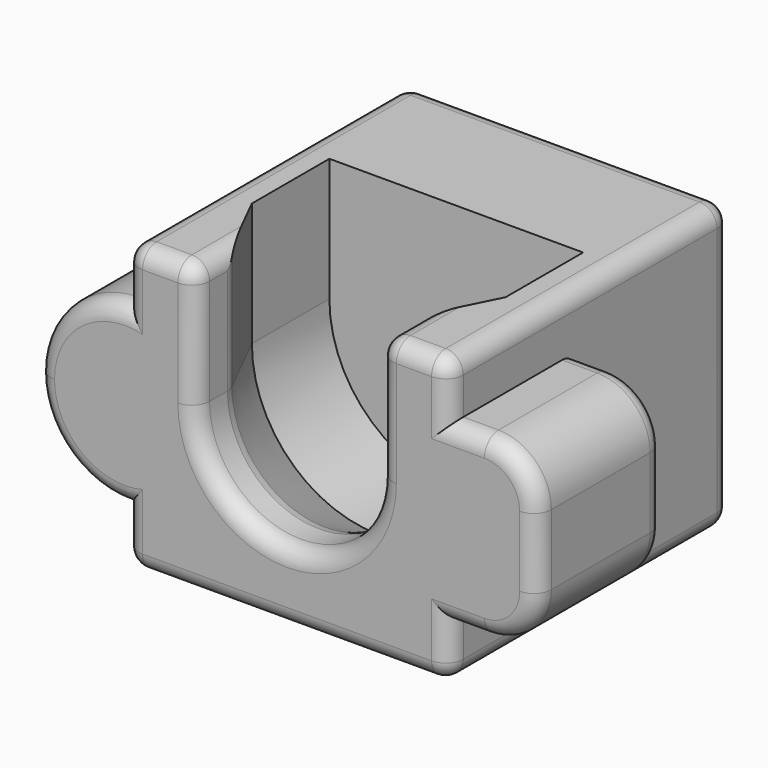
from build123d import *

# Parameters (mm, degrees)
F1_ANGLE = 180
F3_DEPTH = 14
F4_DEPTH = 7
F6_DEPTH = 14
F7_DEPTH = 5
F5_W     = 5
F5_H     = 10
F8_DEPTH = 6
F9_R     = 1


with BuildPart() as f1:
    # F0 (on Top) → F1 (revolve)
    with BuildSketch(Plane.XY):
        Polygon((-9.2, 14), (-9.2, 0), (-5.2, 0), (-5.2, 2.5), (-7.2, 6.5), (-7.2, 12), (0, 12), (0, 14), align=None)
    revolve(axis=Axis((0, -5.2679181099, 0), (0, -1, 0)), revolution_arc=F1_ANGLE)

    # F2 (on face) → F3 (join, through all)
    with BuildSketch(Plane(origin=(0, 14, 0), x_dir=(-1, 0, 0), z_dir=(0, 1, 0))):
        with BuildLine():
            ThreePointArc((-7.9e-09, -9.2), (-6.5053823897, -6.5053823841), (-9.2, 0))
            Line((-9.2, 0), (-9.2, -9.2))
            Line((-9.2, -9.2), (-7.9e-09, -9.2))
        make_face()
        with BuildLine():
            ThreePointArc((9.2, 0), (6.5053823841, -6.5053823897), (-7.9e-09, -9.2))
            Line((-7.9e-09, -9.2), (9.2, -9.2))
            Line((9.2, -9.2), (9.2, 0))
        make_face()
    extrude(amount=-F3_DEPTH)

    # F4 (add): a face of the model
    f4_faces = [f1.faces().sort_by_distance(p)[0] for p in [
        (-8.9687944637, 7, 0),
    ]]
    extrude(f4_faces, amount=F4_DEPTH)

    # F5 (on face) → F6 (join, through all)
    with BuildSketch(Plane(origin=(0, 14, 0), x_dir=(-1, 0, 0), z_dir=(0, 1, 0))):
        with BuildLine():
            ThreePointArc((9.2, -6.1), (12.7355339059, -4.6355339059), (14.2, -1.1))
            ThreePointArc((14.2, -1.1), (12.7355339059, 2.4355339059), (9.2, 3.9))
            Line((9.2, 3.9), (9.2, -6.1))
        make_face()
        with BuildLine():
            Line((-9.2, -6.1), (-9.2, 3.9))
            Line((-9.2, 3.9), (-11.2, 3.9))
            ThreePointArc((-11.2, 3.9), (-13.3213203436, 3.0213203436), (-14.2, 0.9))
            Line((-14.2, 0.9), (-14.2, -3.1))
            ThreePointArc((-14.2, -3.1), (-13.3213203436, -5.2213203436), (-11.2, -6.1))
            Line((-11.2, -6.1), (-9.2, -6.1))
        make_face()
    extrude(amount=-F6_DEPTH)

    # F5 (on face) → F7 (cut)
    with BuildSketch(Plane(origin=(0, 14, 0), x_dir=(-1, 0, 0), z_dir=(0, 1, 0))):
        with BuildLine():
            ThreePointArc((9.2, -6.1), (12.7355339059, -4.6355339059), (14.2, -1.1))
            ThreePointArc((14.2, -1.1), (12.7355339059, 2.4355339059), (9.2, 3.9))
            Line((9.2, 3.9), (9.2, -6.1))
        make_face()
        with BuildLine():
            Line((-9.2, -6.1), (-9.2, 3.9))
            Line((-9.2, 3.9), (-11.2, 3.9))
            ThreePointArc((-11.2, 3.9), (-13.3213203436, 3.0213203436), (-14.2, 0.9))
            Line((-14.2, 0.9), (-14.2, -3.1))
            ThreePointArc((-14.2, -3.1), (-13.3213203436, -5.2213203436), (-11.2, -6.1))
            Line((-11.2, -6.1), (-9.2, -6.1))
        make_face()
    extrude(amount=-F7_DEPTH, mode=Mode.SUBTRACT)

    # F5 (on face) → F8 (join)
    with BuildSketch(Plane(origin=(0, 14, 0), x_dir=(-1, 0, 0), z_dir=(0, 1, 0))):
        with BuildLine():
            Line((9.2, -6.1), (9.2, 3.9))
            ThreePointArc((9.2, 3.9), (4.2, -1.1), (9.2, -6.1))
        make_face()
        with BuildLine():
            ThreePointArc((9.2, -6.1), (4.2, -1.1), (9.2, 3.9))
            Line((9.2, 3.9), (9.2, 7))
            Line((9.2, 7), (-9.2, 7))
            Line((-9.2, 7), (-9.2, 3.9))
            Line((-9.2, 3.9), (-4.2, 3.9))
            Line((-4.2, 3.9), (-4.2, -6.1))
            Line((-4.2, -6.1), (-9.2, -6.1))
            Line((-9.2, -6.1), (-9.2, -9.2))
            Line((-9.2, -9.2), (9.2, -9.2))
            Line((9.2, -9.2), (9.2, -6.1))
        make_face()
        with Locations((-6.7, -1.1)):
            Rectangle(F5_W, F5_H)
    extrude(amount=F8_DEPTH)

    # F9
    f9_edges = [f1.edges().sort_by_distance(p)[0] for p in [
        (9.2, 10, 7),
        (-9.2, 10, 7),
        (9.2, 10, -9.2),
        (-9.2, 10, -9.2),
        (-7.2, 0, 7),
        (9.2, 0, 5.45),
        (9.2, 0, -7.65),
        (-9.2, 0, -7.65),
        (-9.2, 0, 5.45),
        (0, 0, -9.2),
        (0, 0, -5.2),
        (-5.2, 0, 3.5),
        (-14.2, 0, -1.1),
        (10.2, 0, -6.1),
        (13.32132, 0, -5.22132),
        (14.2, 0, -1.1),
        (13.32132, 0, 3.02132),
        (10.2, 0, 3.9),
        (7.2, 0, 7),
        (5.2, 0, 3.5),
        (0, 20, 7),
        (9.2, 20, -1.1),
        (0, 20, -9.2),
        (-9.2, 20, -1.1),
        (-14.2, 9, -1.1),
        (14.2, 9, -1.1),
        (-5.2, 2.5, 3.5),
        (-5.2, 1.25, 7),
        (5.2, 1.25, 7),
        (10.2, 9, -6.1),
        (13.32132, 9, -5.22132),
        (13.32132, 9, 3.02132),
        (10.2, 9, 3.9),
        (5.2, 2.5, 3.5),
        (0, 2.5, -5.2),
    ]]
    fillet(f9_edges, radius=F9_R)


solid = f1.part
